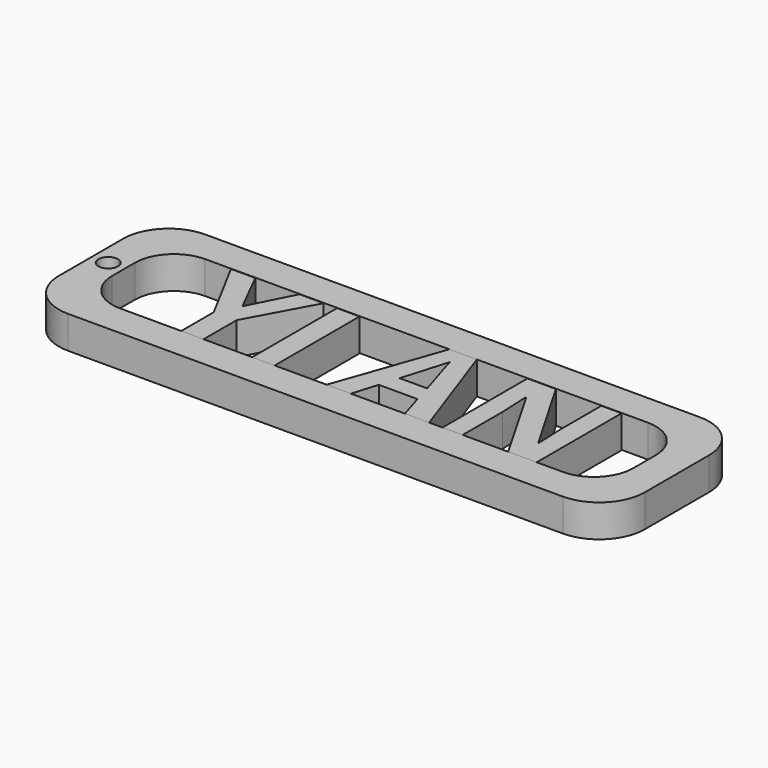
from build123d import *

# Parameters (mm, degrees)
F0_TEXT_SIZE = 22.8299643282
F1_DEPTH     = 5
F2_W         = 90
F2_H         = 26.3662306778
F2_W_2       = 80
F2_H_2       = 16.3662306778
F3_DEPTH     = 5
F4_R         = 7
F5_R         = 6
F6_R         = 1.5
F7_DEPTH     = 5.0010001


# Not quite as in the source:
# - Text() gives the source's letters only with a copy of the font that has no kerning and outlines rounded to 1/6400 em; it was checked with that copy


with BuildPart() as f1:
    # F0 (on Top) → F1 (new body)
    with BuildSketch(Plane.XY):
        with Locations((0, -16.4375743163)):
            Text('YI AN', F0_TEXT_SIZE, font='Open Sans', font_style=FontStyle.BOLD, text_align=(TextAlign.LEFT, TextAlign.BOTTOM))
    extrude(amount=-F1_DEPTH)


with BuildPart() as f3:
    # F2 (on Top) → F3 (new body)
    with BuildSketch(Plane.XY):
        with Locations((30, -8.2544589774)):
            Rectangle(F2_W, F2_H)
        with Locations((30, -8.2544589774)):
            Rectangle(F2_W_2, F2_H_2, mode=Mode.SUBTRACT)
    extrude(amount=-F3_DEPTH)

    # F4
    f4_edges = [f3.edges().sort_by_distance(p)[0] for p in [
        (-15, 4.928656, -2.5),
        (-15, -21.437574, -2.5),
        (75, 4.928656, -2.5),
        (75, -21.437574, -2.5),
    ]]
    fillet(f4_edges, radius=F4_R)

    # F5
    f5_edges = [f3.edges().sort_by_distance(p)[0] for p in [
        (-10, -0.071344, -2.5),
        (-10, -16.437574, -2.5),
        (70, -0.071344, -2.5),
        (70, -16.437574, -2.5),
    ]]
    fillet(f5_edges, radius=F5_R)

    # F6 (on face) → F7 (cut, through all)
    with BuildSketch(Plane.XY):
        with Locations((-12.5, -8.0713436385)):
            Circle(F6_R)
    extrude(amount=-F7_DEPTH, mode=Mode.SUBTRACT)


solid = Compound([f1.part, f3.part])
